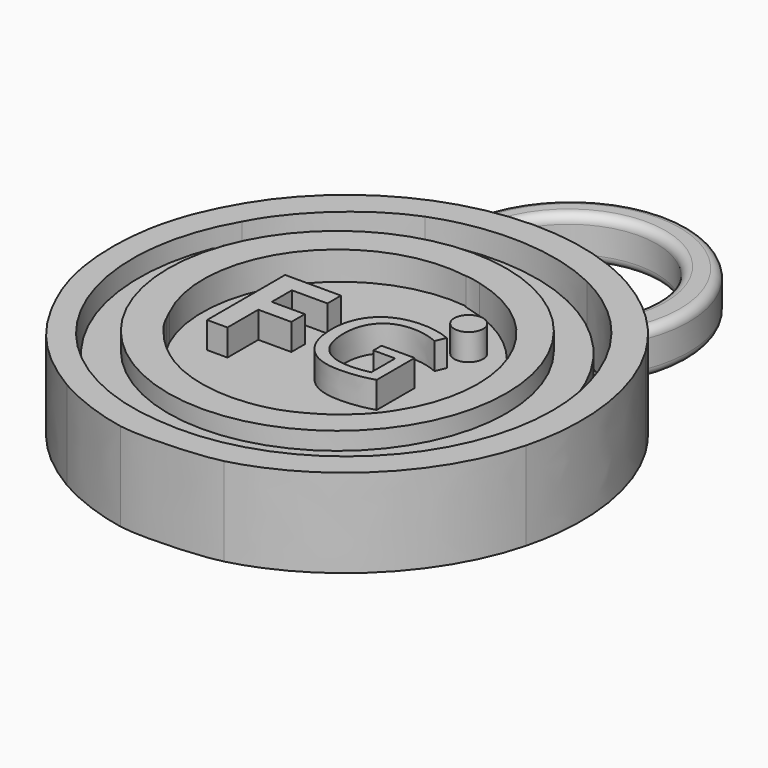
from build123d import *

# Parameters (mm, degrees)
F1_DEPTH     = 7
F0_R         = 19.1279803991
F2_DEPTH     = 10
F3_DEPTH     = 8
F4_DEPTH     = 10
F5_DEPTH     = 5
F6_R         = 1.637802748
F6_TEXT_SIZE = 15.4476677481
F7_DEPTH     = 3
F8_R         = 25.6523292118
F9_DEPTH     = 2
F10_R        = 1


# Not quite as in the source:
# - ends of sketch curves that miss each other by under 0.0002 mm in the source are joined
# - Text() gives the source's letters only with a copy of the font that has no kerning and outlines rounded to 1/6400 em; it was checked with that copy


with BuildPart() as f1:
    # F0 (on Top) → F1 (new body)
    with BuildSketch(Plane.XY):
        with BuildLine():
            ThreePointArc((-59.2347954449, -6.6814816572), (-58.8341384592, -7.4289203643), (-58.392389, -8.152832))
            add(Edge.make_bspline(
                [(-53.744252573, -12.7362436448), (-55.4325929195, -11.5891561276), (-56.9948624064, -10.0566206788), (-58.392389, -8.152832)],
                knots=[0.6895887738, 0.6895887738, 0.6895887738, 0.6895887738, 1, 1, 1, 1], degree=3))
            ThreePointArc((-53.744252573, -12.7362436448), (-41.8918676364, -14.5976951318), (-32.3863979152, -7.277170854))
            add(Edge.make_bspline(
                [(-31.7292377779, -5.9498852292), (-31.9282672637, -6.3926584279), (-32.1497491558, -6.8396976677), (-32.3863979152, -7.277170854)],
                knots=[0.3344487947, 0.3344487947, 0.3344487947, 0.3344487947, 0.5301452615, 0.5301452615, 0.5301452615, 0.5301452615], degree=3))
            ThreePointArc((-31.7292377779, -5.9498852292), (-31.1257115517, -4.3145190756), (-30.7135409768, -2.6207712256))
            add(Edge.make_bspline(
                [(-30.960104, 3.756096), (-30.5099847308, 2.24037654), (-30.4258381475, -0.5496711887), (-30.7135409768, -2.6207712256)],
                knots=[0, 0, 0, 0, 0.8296456494, 0.8296456494, 0.8296456494, 0.8296456494], degree=3))
            add(Edge.make_bspline(
                [(-42.081192, 14.696398), (-36.917409, 13.446373), (-32.566826, 9.166513), (-30.960104, 3.756096)],
                knots=[0, 0, 0, 0, 1, 1, 1, 1], degree=3))
            add(Edge.make_bspline(
                [(-43.101174, 15.090313), (-43.392217, 15.079888), (-42.933225, 14.902656), (-42.081192, 14.696398)],
                knots=[0, 0, 0, 0, 1, 1, 1, 1], degree=3))
            ThreePointArc((-43.101174, 15.090313), (-57.4988268935, 8.8957795494), (-59.2347954449, -6.6814816572))
        make_face()
    extrude(amount=F1_DEPTH)

    # F6 (on face) → F7 (join)
    with BuildSketch(Plane.XY.offset(7)):
        with Locations((-37.2399128973, 8.1431278959)):
            Circle(F6_R)
        with Locations((-57.1012012661, -5.7597728446)):
            Text('F', F6_TEXT_SIZE, font='Open Sans', font_style=FontStyle.BOLD, text_align=(TextAlign.LEFT, TextAlign.BOTTOM))
        with Locations((-46.9719469547, -5.7597728446)):
            Text('G', F6_TEXT_SIZE, font='Open Sans', text_align=(TextAlign.LEFT, TextAlign.BOTTOM))
    extrude(amount=F7_DEPTH)


with BuildPart() as f2:
    # F0 (on Top) → F2 (new body)
    with BuildSketch(Plane.XY):
        with Locations((-45.431247359, -0.1970263361)):
            Circle(F0_R)
        with BuildLine():
            add(Edge.make_bspline(
                [(-41.147337, -15.539034), (-40.1428314806, -15.2993293025), (-39.1027725479, -14.8952129249), (-38.0875846116, -14.3702912296)],
                knots=[0, 0, 0, 0, 0.285965646, 0.285965646, 0.285965646, 0.285965646], degree=3))
            add(Edge.make_bspline(
                [(-52.986997, -13.79839), (-49.483332, -15.87997), (-45.209277, -16.508342), (-41.147337, -15.539034)],
                knots=[0, 0, 0, 0, 1, 1, 1, 1], degree=3))
            add(Edge.make_bspline(
                [(-54.0793245154, -13.0384975043), (-53.6924434387, -13.339610116), (-53.3216500313, -13.5995661142), (-52.986997, -13.79839)],
                knots=[0.8132111093, 0.8132111093, 0.8132111093, 0.8132111093, 1, 1, 1, 1], degree=3))
            ThreePointArc((-54.0793245154, -13.0384975043), (-55.735609132, -11.6635433803), (-57.1866886767, -10.073529))
            add(Edge.make_bspline(
                [(-58.392389, -8.413794), (-58.1519740861, -8.8735062913), (-57.7207609953, -9.4559514121), (-57.1866886767, -10.073529)],
                knots=[0, 0, 0, 0, 0.3057410823, 0.3057410823, 0.3057410823, 0.3057410823], degree=3))
            add(Edge.make_bspline(
                [(-58.730261245, -7.7186027323), (-58.7590058786, -7.7096582658), (-58.6463817969, -7.9281163541), (-58.392389, -8.413794)],
                knots=[0.4434144709, 0.4434144709, 0.4434144709, 0.4434144709, 1, 1, 1, 1], degree=3))
            ThreePointArc((-58.730261245, -7.7186027323), (-58.9921231301, -7.2047098246), (-59.2347954449, -6.6814816572))
            ThreePointArc((-59.2347954449, -6.6814816572), (-57.8562618863, 9.1606507259), (-43.101174, 15.090313))
            add(Edge.make_bspline(
                [(-41.2900061196, 14.7616276316), (-42.0586788101, 14.9772767935), (-42.7191122675, 15.1039614431), (-43.101174, 15.090313)],
                knots=[0.5637105418, 0.5637105418, 0.5637105418, 0.5637105418, 1, 1, 1, 1], degree=3))
            ThreePointArc((-41.2900061196, 14.7616276316), (-32.7178835258, 9.2472094074), (-29.3856387082, -0.3853519649))
            ThreePointArc((-29.3856387082, -0.3853519649), (-30.0245415783, -4.8024790433), (-31.888879, -8.857532))
            add(Edge.make_bspline(
                [(-33.6493462178, -11.097555272), (-32.9505648152, -10.3812991178), (-32.3492889696, -9.624194109), (-31.888879, -8.857532)],
                knots=[0.7439800073, 0.7439800073, 0.7439800073, 0.7439800073, 1, 1, 1, 1], degree=3))
            ThreePointArc((-33.6493462178, -11.097555272), (-35.7226006868, -12.9317340256), (-38.0875846116, -14.3702912296))
        make_face(mode=Mode.SUBTRACT)
    extrude(amount=F2_DEPTH)

    # F0 (on Top) → F3 (join)
    with BuildSketch(Plane.XY):
        with BuildLine():
            Line((-47.069925, -23.475932), (-44.027216, -23.25211))
            add(Edge.make_bspline(
                [(-30.1205396487, -17.7460547966), (-33.8374032042, -20.9263141883), (-38.6163066312, -22.8540931532), (-44.027216, -23.25211)],
                knots=[0.3732264922, 0.3732264922, 0.3732264922, 0.3732264922, 1, 1, 1, 1], degree=3))
            ThreePointArc((-30.1205396487, -17.7460547966), (-24.6034613901, -10.3216274381), (-22.479647618, -1.3188673516))
            add(Edge.make_bspline(
                [(-22.475115, -0.230342), (-22.4741181138, -0.6104670398), (-22.4754785569, -0.9725951682), (-22.479647618, -1.3188673516)],
                knots=[0, 0, 0, 0, 0.0758203688, 0.0758203688, 0.0758203688, 0.0758203688], degree=3))
            ThreePointArc((-22.475115, -0.230342), (-34.5455591496, 19.4779960315), (-57.639349598, 18.5885846227))
            add(Edge.make_bspline(
                [(-63.906497, 12.228838), (-62.4986856864, 14.3385524124), (-59.8791359743, 16.9840424416), (-57.639349598, 18.5885846227)],
                knots=[0, 0, 0, 0, 0.9296926806, 0.9296926806, 0.9296926806, 0.9296926806], degree=3))
            add(Edge.make_bspline(
                [(-65.056999, 10.88216), (-65.696203, 9.619423), (-65.474943, 9.878406), (-63.906497, 12.228838)],
                knots=[0, 0, 0, 0, 1, 1, 1, 1], degree=3))
            ThreePointArc((-65.056999, 10.88216), (-65.4973944672, 10.0234562282), (-65.9020070893, 9.1473232695))
            add(Edge.make_bspline(
                [(-65.731153, 9.162373), (-65.731153, 9.2769531771), (-65.8027128579, 9.2644038713), (-65.9020070893, 9.1473232695)],
                knots=[0, 0, 0, 0, 0.7874114494, 0.7874114494, 0.7874114494, 0.7874114494], degree=3))
            add(Edge.make_bspline(
                [(-65.987633, 8.500911), (-65.846569, 8.719191), (-65.731153, 9.016851), (-65.731153, 9.162373)],
                knots=[0, 0, 0, 0, 1, 1, 1, 1], degree=3))
            add(Edge.make_bspline(
                [(-66.2406641823, 8.3307092691), (-66.2205050198, 8.2367620574), (-66.1144310132, 8.3047064339), (-65.987633, 8.500911)],
                knots=[0.10113768, 0.10113768, 0.10113768, 0.10113768, 1, 1, 1, 1], degree=3))
            ThreePointArc((-66.2406641823, 8.3307092691), (-64.5014500877, -12.3017054982), (-47.069925, -23.475932))
        make_face()
        with Locations((-45.431247359, -0.1970263361)):
            Circle(F0_R, mode=Mode.SUBTRACT)
    extrude(amount=F3_DEPTH)


with BuildPart() as f4:
    # F0 (on Top) → F4 (new body)
    with BuildSketch(Plane.XY):
        with BuildLine():
            add(Edge.make_bspline(
                [(-48.970073, -26.413517), (-51.625486, -25.940057), (-55.306082, -24.572912), (-57.588797, -23.212105)],
                knots=[0, 0, 0, 0, 1, 1, 1, 1], degree=3))
            add(Edge.make_bspline(
                [(-37.677216, -25.917347), (-40.204587, -26.574122), (-46.514432, -26.851352), (-48.970073, -26.413517)],
                knots=[0, 0, 0, 0, 1, 1, 1, 1], degree=3))
            add(Edge.make_bspline(
                [(-18.723931, -6.903355), (-21.072064, -16.0174), (-28.585257, -23.554652), (-37.677216, -25.917347)],
                knots=[0, 0, 0, 0, 1, 1, 1, 1], degree=3))
            add(Edge.make_bspline(
                [(-21.637296, 13.639865), (-17.980309, 7.51172), (-16.925794, 0.075943), (-18.723931, -6.903355)],
                knots=[0, 0, 0, 0, 1, 1, 1, 1], degree=3))
            ThreePointArc((-21.637296, 13.639865), (-25.8109452117, 18.893261801), (-31.164960657, 22.9370279049))
            ThreePointArc((-31.164960657, 22.9370279049), (-32.8667693195, 23.8327160783), (-34.6287693504, 24.6032781578))
            ThreePointArc((-34.6287693504, 24.6032781578), (-43.3302550234, 26.4435054284), (-52.1524980847, 25.3164221611))
            ThreePointArc((-52.1524980847, 25.3164221611), (-59.7026840443, 21.640329328), (-65.733156707, 15.7963267608))
            add(Edge.make_bspline(
                [(-69.2860531049, 9.3594504448), (-68.3414214755, 11.7099431853), (-67.1463052527, 13.8651148137), (-65.733156707, 15.7963267608)],
                knots=[0.0254254095, 0.0254254095, 0.0254254095, 0.0254254095, 0.2859602016, 0.2859602016, 0.2859602016, 0.2859602016], degree=3))
            ThreePointArc((-69.2860531049, 9.3594504448), (-69.4192204262, 9.0043367676), (-69.547318, 8.647363))
            ThreePointArc((-69.547318, 8.647363), (-70.144466641, 6.7128124545), (-70.5929494637, 4.7384934654))
            add(Edge.make_bspline(
                [(-69.40493, -9.153827), (-71.00351631, -5.1220863609), (-71.4043965437, 0.1179787787), (-70.5929494637, 4.7384934654)],
                knots=[0, 0, 0, 0, 0.7708246728, 0.7708246728, 0.7708246728, 0.7708246728], degree=3))
            add(Edge.make_bspline(
                [(-57.588797, -23.212105), (-63.292625, -19.811874), (-66.863546, -15.563365), (-69.40493, -9.153827)],
                knots=[0, 0, 0, 0, 1, 1, 1, 1], degree=3))
        make_face()
        with BuildLine():
            ThreePointArc((-21.0622935478, -0.2228973471), (-28.8652464336, -17.66638119), (-47.069925, -23.475932))
            ThreePointArc((-47.069925, -23.475932), (-65.5880574373, -11.2831815996), (-65.056999, 10.88216))
            add(Edge.make_bspline(
                [(-53.02305, 21.71414), (-57.817765, 19.865098), (-62.763129, 15.413691), (-65.056999, 10.88216)],
                knots=[0, 0, 0, 0, 1, 1, 1, 1], degree=3))
            add(Edge.make_bspline(
                [(-34.119623, 20.950198), (-39.888503, 23.76455), (-46.964626, 24.050518), (-53.02305, 21.71414)],
                knots=[0, 0, 0, 0, 1, 1, 1, 1], degree=3))
            add(Edge.make_bspline(
                [(-21.879548, 5.907178), (-23.680713, 12.54305), (-28.152859, 18.039306), (-34.119623, 20.950198)],
                knots=[0, 0, 0, 0, 1, 1, 1, 1], degree=3))
            ThreePointArc((-21.879548, 5.907178), (-21.2675070442, 2.8692592062), (-21.0622935478, -0.2228973471))
        make_face(mode=Mode.SUBTRACT)
    extrude(amount=F4_DEPTH)


with BuildPart() as f5:
    # F0 (on Top) → F5 (new body)
    with BuildSketch(Plane.XY):
        with BuildLine():
            add(Edge.make_bspline(
                [(-34.5666196684, 24.7092430798), (-33.3810366932, 24.2207005987), (-32.2320034389, 23.6484291155), (-31.1295313761, 23.0001864934)],
                knots=[0.1322045887, 0.1322045887, 0.1322045887, 0.1322045887, 0.3238140526, 0.3238140526, 0.3238140526, 0.3238140526], degree=3))
            ThreePointArc((-31.1295313761, 23.0001864934), (-42.0731684167, 42.8839416727), (-55.1710537864, 24.3482380025))
            add(Edge.make_bspline(
                [(-55.1710537864, 24.3482380025), (-54.2149744978, 24.769792958), (-53.2281255532, 25.1355815735), (-52.2133910902, 25.4430586472)],
                knots=[0.7959745665, 0.7959745665, 0.7959745665, 0.7959745665, 0.9122414491, 0.9122414491, 0.9122414491, 0.9122414491], degree=3))
            ThreePointArc((-52.2133910902, 25.4430586472), (-42.7834765104, 39.6619361545), (-34.5666196684, 24.7092430798))
        make_face()
    extrude(amount=F5_DEPTH)

    # F10
    f10_edges = [f5.edges().sort_by_distance(p)[0] for p in [
        (-42.783477, 39.661936, 5),
        (-42.073168, 42.883942, 5),
        (-42.073168, 42.883942, 0),
        (-42.783477, 39.661936, 0),
    ]]
    fillet(f10_edges, radius=F10_R)


with BuildPart() as f9:
    # F8 (on Top) → F9 (new body)
    with BuildSketch(Plane.XY):
        with Locations((-44.544095667, -0.2898088063)):
            Circle(F8_R)
    extrude(amount=F9_DEPTH)


solid = Compound([f1.part, f2.part, f4.part, f5.part, f9.part])
